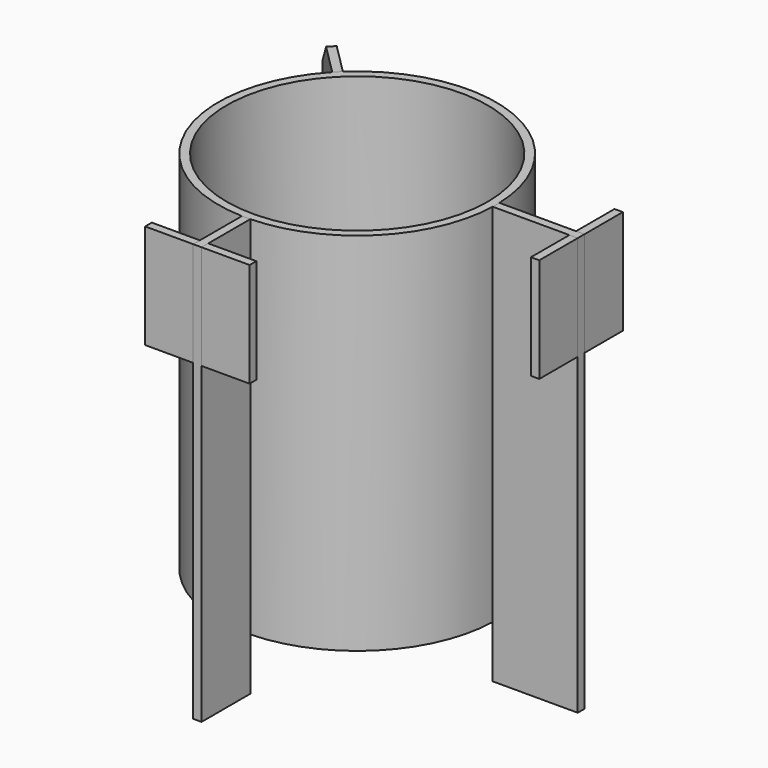
from build123d import *

# Parameters (mm, degrees)
F1_DEPTH = 80
F0_W     = 1.6
F0_H     = 1.6
F0_R     = 25
F2_DEPTH = 70
F3_SIZE  = 5
F0_W_2   = 9.2
F4_DEPTH = 20
F0_H_2   = 9.2


with BuildPart() as f1:
    # F0 (on Top) → F1 (new body)
    with BuildSketch(Plane.XY):
        with BuildLine():
            ThreePointArc((-34.1844936712, 30.2744241403), (-33.6273167185, 30.8486180375), (-33.0531228213, 31.4057949902))
            Line((-33.0531228213, 31.4057949902), (-42.4661514833, 40.8188236522))
            Line((-42.4661514833, 40.8188236522), (-43.5975223332, 39.6874528023))
            Line((-43.5975223332, 39.6874528023), (-34.1844936712, 30.2744241403))
        make_face()
    extrude(amount=-F1_DEPTH)

    # F3
    f3_edges = [f1.edges().sort_by_distance(p)[0] for p in [
        (-43.031837, 40.253138, -80),
        (-43.031837, 40.253138, 0),
    ]]
    chamfer(f3_edges, length=F3_SIZE)


with BuildPart() as f1b:
    # F0 (on Top) → F1, piece 2 (new body)
    with BuildSketch(Plane.XY):
        with BuildLine():
            Line((-14.0182763389, -24.6038896912), (-14.0182763389, -14.5483895453))
            ThreePointArc((-14.0182763389, -14.5483895453), (-14.8182763389, -14.5604223421), (-15.6182763389, -14.5483895453))
            Line((-15.6182763389, -14.5483895453), (-15.6182763389, -24.6038896912))
            Line((-15.6182763389, -24.6038896912), (-14.0182763389, -24.6038896912))
        make_face()
        with Locations((-14.8182763389, -25.4038896912)):
            Rectangle(F0_W, F0_H)
    extrude(amount=-F1_DEPTH)


with BuildPart() as f1c:
    # F0 (on Top) → F1, piece 3 (new body)
    with BuildSketch(Plane.XY):
        with BuildLine():
            ThreePointArc((11.7696908643, 12.8395776579), (11.7787152918, 12.4396229017), (11.7817236611, 12.0395776579))
            ThreePointArc((11.7817236611, 12.0395776579), (11.7787152918, 11.6395324142), (11.7696908643, 11.2395776579))
            Line((11.7696908643, 11.2395776579), (26.4436644382, 11.2395776579))
            Line((26.4436644382, 11.2395776579), (26.4436644382, 12.8395776579))
            Line((26.4436644382, 12.8395776579), (11.7696908643, 12.8395776579))
        make_face()
        with Locations((27.2436644382, 12.0395776579)):
            Rectangle(F0_W, F0_H)
    extrude(amount=-F1_DEPTH)


with BuildPart() as f2:
    # F0 (on Top) → F2 (new body)
    with BuildSketch(Plane.XY):
        with BuildLine():
            ThreePointArc((11.7696908643, 11.2395776579), (11.7787152918, 11.6395324142), (11.7817236611, 12.0395776579))
            ThreePointArc((11.7817236611, 12.0395776579), (11.7787152918, 12.4396229017), (11.7696908643, 12.8395776579))
            ThreePointArc((11.7696908643, 12.8395776579), (-4.638897038, 36.6147732227), (-33.0531228213, 31.4057949902))
            ThreePointArc((-33.0531228213, 31.4057949902), (-33.6273167185, 30.8486180375), (-34.1844936712, 30.2744241403))
            ThreePointArc((-34.1844936712, 30.2744241403), (-39.3934719037, 1.860198357), (-15.6182763389, -14.5483895453))
            ThreePointArc((-15.6182763389, -14.5483895453), (-14.8182763389, -14.5604223421), (-14.0182763389, -14.5483895453))
            ThreePointArc((-14.0182763389, -14.5483895453), (3.9907640406, -6.7694627217), (11.7696908643, 11.2395776579))
        make_face()
        with Locations((-14.8182763389, 12.0395776579)):
            Circle(F0_R, mode=Mode.SUBTRACT)
    extrude(amount=-F2_DEPTH)


with BuildPart() as f4:
    # F0 (on Top) → F4 (new body)
    with BuildSketch(Plane.XY):
        with Locations((-20.2182763389, -25.4038896912)):
            Rectangle(F0_W_2, F0_H)
    extrude(amount=-F4_DEPTH)


with BuildPart() as f4b:
    # F0 (on Top) → F4, piece 2 (new body)
    with BuildSketch(Plane.XY):
        with Locations((-9.4182763389, -25.4038896912)):
            Rectangle(F0_W_2, F0_H)
    extrude(amount=-F4_DEPTH)


with BuildPart() as f4c:
    # F0 (on Top) → F4, piece 3 (new body)
    with BuildSketch(Plane.XY):
        with Locations((27.2436644382, 6.6395776579)):
            Rectangle(F0_W, F0_H_2)
    extrude(amount=-F4_DEPTH)


with BuildPart() as f4d:
    # F0 (on Top) → F4, piece 4 (new body)
    with BuildSketch(Plane.XY):
        with Locations((27.2436644382, 17.4395776579)):
            Rectangle(F0_W, F0_H_2)
    extrude(amount=-F4_DEPTH)


solid = Compound([f1.part, f1b.part, f1c.part, f2.part, f4.part, f4b.part, f4c.part, f4d.part])
